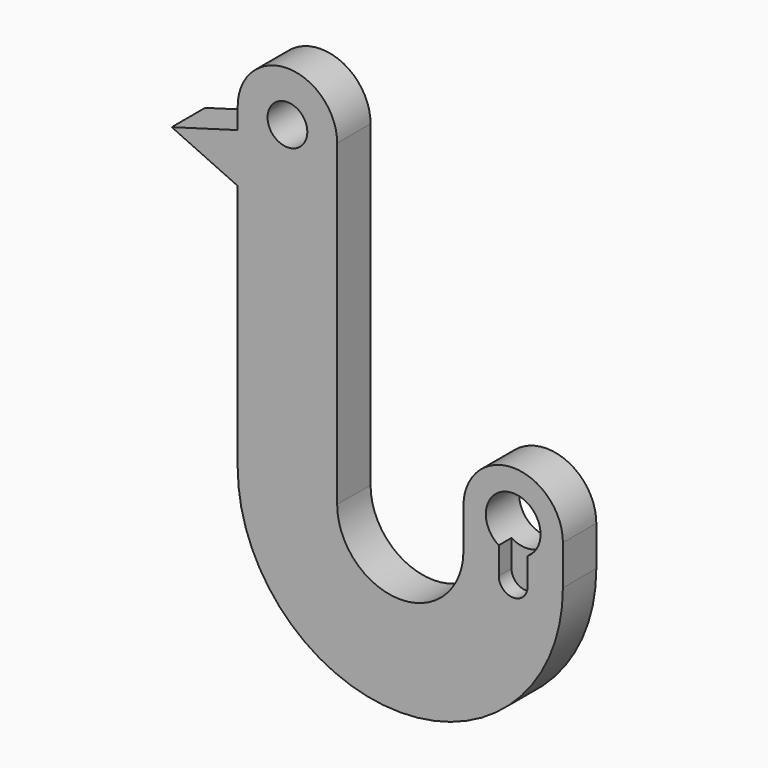
from build123d import *

# Parameters (mm, degrees)
F1_R     = 2.75
F1_R_2   = 2
F2_DEPTH = 4.2
F4_DEPTH = 1.6


with BuildPart() as f2:
    # F1 (on Front) → F2 (new body)
    with BuildSketch(Plane.XZ):
        with BuildLine():
            Line((-6.3493797847, -4), (-6.3493798562, 27.98366989))
            ThreePointArc((-6.3493798562, 27.98366989), (-11.3493798562, 32.9836699012), (-16.3493798562, 27.98366989))
            Line((-16.3493798562, 27.98366989), (-16.3493798515, 25.8790112235))
            Line((-16.3493798515, 25.8790112235), (-22.9881312178, 23.98366989))
            Line((-22.9881312178, 23.98366989), (-16.3493798405, 20.9362090031))
            Line((-16.3493798405, 20.9362090031), (-16.3493797847, -4))
            ThreePointArc((-16.3493797847, -4), (0, -20.349379785), (16.3493797847, -4))
            Line((16.3493797847, -4), (16.3493797847, 0))
            ThreePointArc((16.3493797847, 0), (11.3493797847, 5), (6.3493797847, 0))
            Line((6.3493797847, 0), (6.3493797847, -4))
            ThreePointArc((6.3493797847, -4), (0, -10.3493797847), (-6.3493797847, -4))
        make_face()
        with Locations((11.3493797847, 0)):
            Circle(F1_R, mode=Mode.SUBTRACT)
        with Locations((-11.3493798562, 27.9836699012)):
            Circle(F1_R_2, mode=Mode.SUBTRACT)
    extrude(amount=F2_DEPTH)

    # F3 (on face) → F4 (cut)
    with BuildSketch(Plane.XZ.offset(4.2)):
        with BuildLine():
            ThreePointArc((9.8993797847, -2.3366642891), (11.3493797847, -2.75), (12.7993797847, -2.3366642891))
            ThreePointArc((12.7993797847, -2.3366642891), (13.7525027528, -1.3369741957), (14.0993797847, 0))
            ThreePointArc((14.0993797847, 0), (10.012405589, 2.4031229681), (9.8993797847, -2.3366642891))
        make_face()
        with BuildLine():
            Line((12.7993797847, -5.05), (12.7993797847, -2.3366642891))
            ThreePointArc((12.7993797847, -2.3366642891), (11.3493797847, -2.75), (9.8993797847, -2.3366642891))
            Line((9.8993797847, -2.3366642891), (9.8993797847, -5.05))
            ThreePointArc((9.8993797847, -5.05), (11.3493797847, -6.5), (12.7993797847, -5.05))
        make_face()
    extrude(amount=-F4_DEPTH, mode=Mode.SUBTRACT)


solid = f2.part
